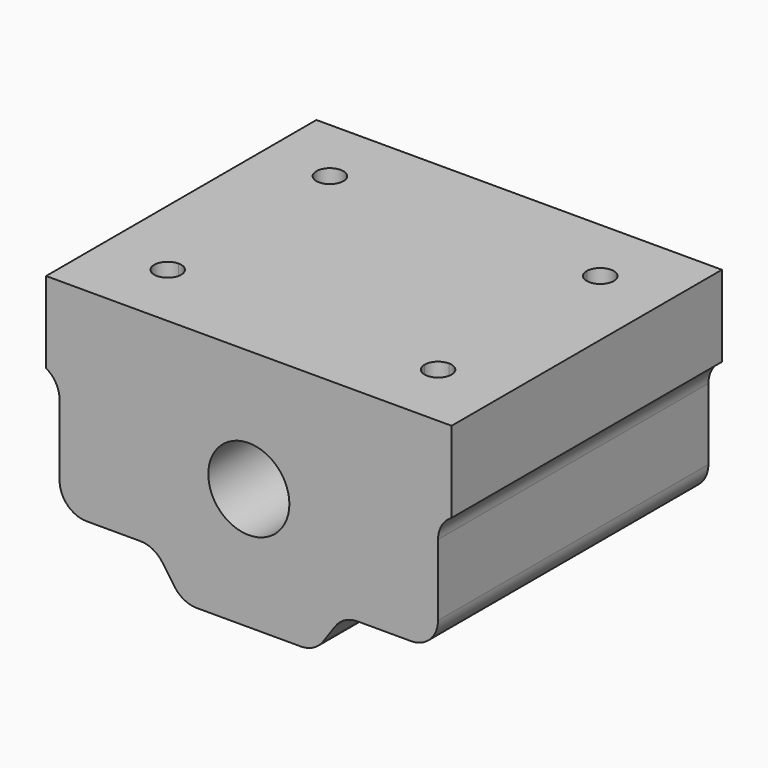
from build123d import *

# Parameters (mm, degrees)
F0_R         = 3
F1_DEPTH     = 25
F3_DEPTH     = 18.001
F4_T1_DEPTH  = 25
F4_T3_DEPTH  = 25
F4_T5_DEPTH  = 25
F4_T7_DEPTH  = 25
F4_T9_DEPTH  = 35
F4_T11_DEPTH = 30.1931758285
F4_T13_DEPTH = 30.1931758285
F4_T15_DEPTH = 35


# Not quite as in the source:
# - a fillet or chamfer that OpenCascade refuses, or shapes differently, is made with other operations: its cross-section is extruded or revolved along the edge and cut away or added


with BuildPart() as f1:
    # F0 (on Front) → F1 (new body)
    with BuildSketch(Plane.XZ):
        Polygon((15, 9), (-15, 9), (-15, 3), (-14, 3), (-14, -6), (-7, -6), (-4.890570417, -9), (4.890570417, -9), (7, -6), (14, -6), (14, 3), (15, 3), align=None)
        Circle(F0_R, mode=Mode.SUBTRACT)
    extrude(amount=F1_DEPTH)

    # F2 (on face) → F3 (cut, through all)
    with BuildSketch(Plane.XY.offset(9)):
        with BuildLine():
            Line((10, -5), (10, -6))
            ThreePointArc((10, -6), (10.7071067812, -5.7071067812), (11, -5))
            ThreePointArc((11, -5), (10, -4), (9, -5))
            Line((9, -5), (10, -5))
        make_face()
        with BuildLine():
            ThreePointArc((9, -5), (9.2928932188, -5.7071067812), (10, -6))
            Line((10, -6), (10, -5))
            Line((10, -5), (9, -5))
        make_face()
        with BuildLine():
            Line((10, -20), (9, -20))
            ThreePointArc((9, -20), (10, -21), (11, -20))
            ThreePointArc((11, -20), (10.7071067812, -19.2928932188), (10, -19))
            Line((10, -19), (10, -20))
        make_face()
        with BuildLine():
            ThreePointArc((10, -19), (9.2928932188, -19.2928932188), (9, -20))
            Line((9, -20), (10, -20))
            Line((10, -20), (10, -19))
        make_face()
        with BuildLine():
            ThreePointArc((-10, -19), (-10.7071067812, -20.7071067812), (-9, -20))
            Line((-9, -20), (-10, -20))
            Line((-10, -20), (-10, -19))
        make_face()
        with BuildLine():
            Line((-10, -20), (-9, -20))
            ThreePointArc((-9, -20), (-9.2928932188, -19.2928932188), (-10, -19))
            Line((-10, -19), (-10, -20))
        make_face()
        with BuildLine():
            ThreePointArc((-9, -5), (-10.7071067812, -4.2928932188), (-10, -6))
            Line((-10, -6), (-10, -5))
            Line((-10, -5), (-9, -5))
        make_face()
        with BuildLine():
            Line((-10, -5), (-10, -6))
            ThreePointArc((-10, -6), (-9.2928932188, -5.7071067812), (-9, -5))
            Line((-9, -5), (-10, -5))
        make_face()
    extrude(amount=-F3_DEPTH, mode=Mode.SUBTRACT)

    # F4: fillet of radius 2 on 8 edges, made by hand

    # F4_s2 → F4_t1 (join)
    with BuildSketch(Plane.XZ):
        with BuildLine():
            ThreePointArc((15, 3), (14.2679491924, 2.2679491924), (14, 1.2679491924))
            Line((14, 1.2679491924), (14, 3))
            Line((14, 3), (15, 3))
        make_face()
    extrude(amount=F4_T1_DEPTH)

    # F4_s4 → F4_t3 (join)
    with BuildSketch(Plane.XZ):
        with BuildLine():
            ThreePointArc((-15, 3), (-14.2679491924, 2.2679491924), (-14, 1.2679491924))
            Line((-14, 1.2679491924), (-14, 3))
            Line((-14, 3), (-15, 3))
        make_face()
    extrude(amount=F4_T3_DEPTH)

    # F4_s6 → F4_t5 (join)
    with BuildSketch(Plane.XZ):
        with BuildLine():
            ThreePointArc((-8.0386351657, -6), (-7.1168832592, -6.2250708682), (-6.4025908546, -6.8496265771))
            Line((-6.4025908546, -6.8496265771), (-7, -6))
            Line((-7, -6), (-8.0386351657, -6))
        make_face()
    extrude(amount=F4_T5_DEPTH)

    # F4_s8 → F4_t7 (join)
    with BuildSketch(Plane.XZ):
        with BuildLine():
            ThreePointArc((6.4025908546, -6.8496265771), (7.1168832592, -6.2250708682), (8.0386351657, -6))
            Line((8.0386351657, -6), (7, -6))
            Line((7, -6), (6.4025908546, -6.8496265771))
        make_face()
    extrude(amount=F4_T7_DEPTH)

    # F4_s10 → F4_t9 (cut)
    with BuildSketch(Plane.XZ.offset(-5)):
        with BuildLine():
            ThreePointArc((-14, -4), (-13.4142135624, -5.4142135624), (-12, -6))
            Line((-12, -6), (-14, -6))
            Line((-14, -6), (-14, -4))
        make_face()
    extrude(amount=F4_T9_DEPTH, mode=Mode.SUBTRACT)

    # F4_s12 → F4_t11 (cut)
    with BuildSketch(Plane.XZ.offset(-2.5965879143)):
        with BuildLine():
            ThreePointArc((-3.8519352513, -9), (-4.7736871578, -8.7749291318), (-5.4879795624, -8.1503734229))
            Line((-5.4879795624, -8.1503734229), (-4.890570417, -9))
            Line((-4.890570417, -9), (-3.8519352513, -9))
        make_face()
    extrude(amount=F4_T11_DEPTH, mode=Mode.SUBTRACT)

    # F4_s14 → F4_t13 (cut)
    with BuildSketch(Plane.XZ.offset(-2.5965879143)):
        with BuildLine():
            ThreePointArc((5.4879795624, -8.1503734229), (4.7736871578, -8.7749291318), (3.8519352513, -9))
            Line((3.8519352513, -9), (4.890570417, -9))
            Line((4.890570417, -9), (5.4879795624, -8.1503734229))
        make_face()
    extrude(amount=F4_T13_DEPTH, mode=Mode.SUBTRACT)

    # F4_s16 → F4_t15 (cut)
    with BuildSketch(Plane.XZ.offset(-5)):
        with BuildLine():
            ThreePointArc((14, -4), (13.4142135624, -5.4142135624), (12, -6))
            Line((12, -6), (14, -6))
            Line((14, -6), (14, -4))
        make_face()
    extrude(amount=F4_T15_DEPTH, mode=Mode.SUBTRACT)


solid = f1.part
